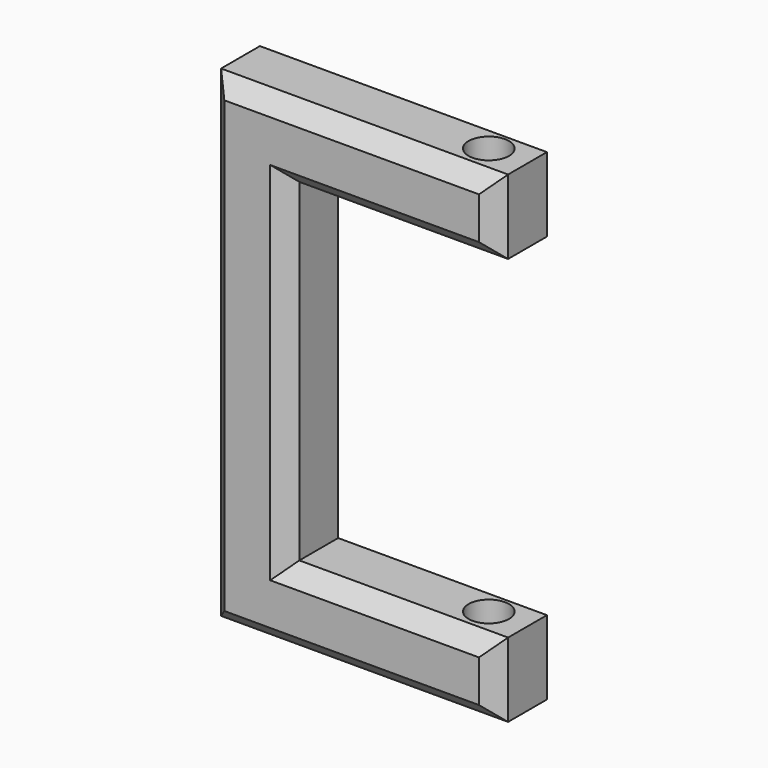
from build123d import *

# Parameters (mm, degrees)
F1_DEPTH = 6.35
F3_D     = 6.35
F4_SIZE  = 2.54
F5_SIZE  = 2.54
F6_SIZE  = 2.53999


# Not quite as in the source:
# - a fillet or chamfer is up to 0.001 mm smaller than in the source, because OpenCascade refuses the exact size


with BuildPart() as f1:
    # F0 (on Front) → F1 (new body, symmetric)
    with BuildSketch(Plane.XZ):
        Polygon((-45.0841039419, 0), (0, 0), (0, 11.6680786014), (-32.7930003405, 11.6680786014), (-32.7930003405, 64.019061625), (0, 64.019061625), (0, 75.703188777), (-45.0841039419, 75.703188777), align=None)
    extrude(amount=F1_DEPTH, both=True)

    # F3 (through all)
    with Locations(Plane(origin=(0, 0, 0), x_dir=(1, 0, 0), z_dir=(0, 0, -1))):
        with Locations((-6.1689345166, -0.1147333004)):
            Hole(F3_D / 2)

    # F4
    f4_edges = [f1.edges().sort_by_distance(p)[0] for p in [
        (-22.542052, -6.35, 75.703189),
        (-22.542052, 6.35, 75.703189),
        (-16.3965, -6.35, 64.019062),
        (0, -6.35, 69.861125),
        (0, 6.35, 69.861125),
        (-16.3965, 6.35, 64.019062),
    ]]
    chamfer(f4_edges, length=F4_SIZE)

    # F5
    f5_edges = [f1.edges().sort_by_distance(p)[0] for p in [
        (-22.542052, 6.35, 0),
        (0, -6.35, 5.834039),
        (-22.542052, -6.35, 0),
        (-16.3965, -6.35, 11.668079),
        (0, 6.35, 5.834039),
        (-16.3965, 6.35, 11.668079),
    ]]
    chamfer(f5_edges, length=F5_SIZE)

    # F6 (size 2.54 in the source; OpenCascade refuses exactly that, so slightly less here)
    f6_edges = [f1.edges().sort_by_distance(p)[0] for p in [
        (-45.084104, 6.35, 37.851594),
        (-32.793, -6.35, 37.84357),
        (-32.793, 6.35, 37.84357),
        (-45.084104, -6.35, 37.851594),
    ]]
    chamfer(f6_edges, length=F6_SIZE)


solid = f1.part
